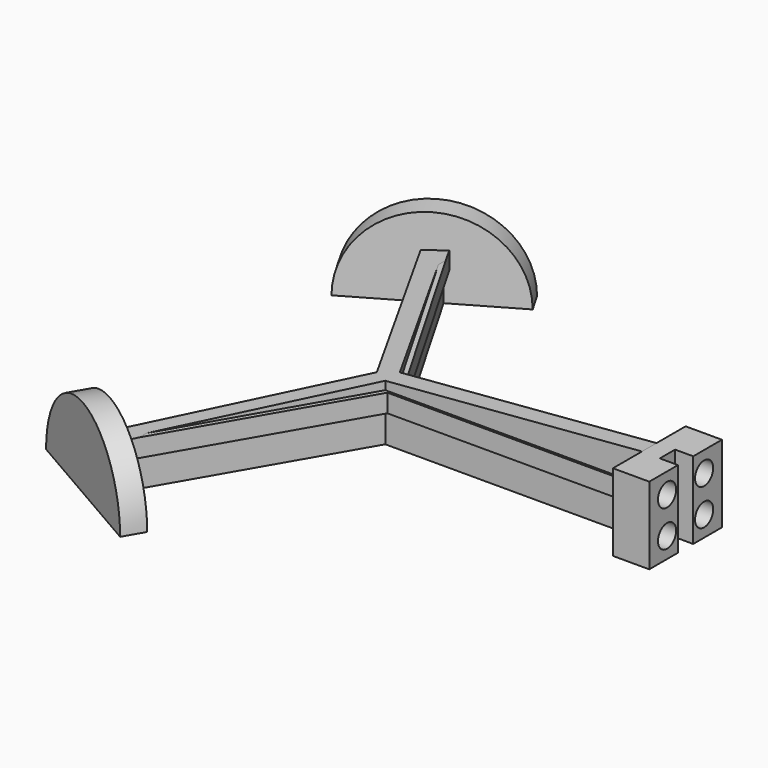
from build123d import *

# Parameters (mm, degrees)
F0_W      = 20
F0_H      = 17
F1_DEPTH  = 8
F2_W      = 4
F2_H      = 4.2
F3_DEPTH  = 17.001
F4_R      = 2.5
F5_DEPTH  = 8.001
F6_W      = 4
F6_H      = 6.5
F6_W_2    = 0.5
F6_H_2    = 4
F7_DEPTH  = 60
F9_DEPTH  = 17.001
F10_DEPTH = 50
F11_DEPTH = 50
F13_DEPTH = 47.8022701892
F14_DEPTH = 43.8022701892
F15_R     = 17.5
F16_DEPTH = 5
F17_R     = 17.5
F18_DEPTH = 5
F20_DEPTH = 108.9243937587


# Not quite as in the source:
# - a feature names something its author has since deleted; it is built from what else it names


with BuildPart() as f1:
    # F0 (on Right) → F1 (new body)
    with BuildSketch(Plane.YZ):
        Rectangle(F0_W, F0_H)
    extrude(amount=F1_DEPTH)

    # F2 (on face) → F3 (cut, through all)
    with BuildSketch(Plane.XY.offset(8.5)):
        with Locations((6, 0)):
            Rectangle(F2_W, F2_H)
    extrude(amount=-F3_DEPTH, mode=Mode.SUBTRACT)

    # F4 (on face) → F5 (cut, through all)
    with BuildSketch(Plane.YZ.offset(8)):
        with Locations((-5.1, 4)):
            Circle(F4_R)
        with Locations((5.1, 4)):
            Circle(F4_R)
        with Locations((-5.1, -4)):
            Circle(F4_R)
        with Locations((5.1, -4)):
            Circle(F4_R)
    extrude(amount=-F5_DEPTH, mode=Mode.SUBTRACT)

    # F6 (on Right) → F7 (join)
    with BuildSketch(Plane.YZ):
        with Locations((0, 5.25)):
            Rectangle(F6_W, F6_H)
        with Locations((2.25, 0)):
            Rectangle(F6_W_2, F6_H_2)
        Rectangle(F6_W, F6_H_2)
        with Locations((-2.25, 0)):
            Rectangle(F6_W_2, F6_H_2)
        with Locations((0, -5.25)):
            Rectangle(F6_W, F6_H)
    extrude(amount=-F7_DEPTH)

    # F8 (on face) → F9 (cut, through all)
    with BuildSketch(Plane.XY.offset(8.5)):
        Polygon((-60, -2.5), (-55.6698729811, -2.5), (-60, 0), align=None)
        Polygon((-60, 2.5), (-60, 0), (-55.6698729811, 2.5), align=None)
    extrude(amount=-F9_DEPTH, mode=Mode.SUBTRACT)

    # F10 (add): a face of the model
    f10_faces = [f1.faces().sort_by_distance(p)[0] for p in [
        (-58.1476678863, -1.0694444444, 0),
    ]]
    extrude(f10_faces, amount=F10_DEPTH)

    # F11 (add): a face of the model
    f11_faces = [f1.faces().sort_by_distance(p)[0] for p in [
        (-58.1476678863, 1.0694444444, 0),
    ]]
    extrude(f11_faces, amount=F11_DEPTH)

    # F12 (on face) → F13 (cut, through all)
    with BuildSketch(Plane.XZ.offset(2)):
        Polygon((0, 8.5), (-90.0749489665, 12.646025978), (-90.0749489665, 1.0502453661), align=None)
    extrude(amount=-F13_DEPTH, mode=Mode.SUBTRACT)

    # F12 (on face) → F14 (cut, through all)
    with BuildSketch(Plane.XZ.offset(2)):
        Polygon((0, 8.5), (-90.0749489665, 12.646025978), (-90.0749489665, 1.0502453661), align=None)
    extrude(amount=F14_DEPTH, mode=Mode.SUBTRACT)

    # F15 (on face) → F16 (join)
    with BuildSketch(Plane(origin=(-40, -69.2820323028, 0), x_dir=(0.8660254038, -0.5, 0), z_dir=(-0.5, -0.8660254038, 0))):
        with Locations((-49.9615242271, -8.5)):
            Circle(F15_R)
    extrude(amount=F16_DEPTH)

    # F17 (on face) → F18 (join)
    with BuildSketch(Plane(origin=(-40, 69.2820323028, 0), x_dir=(-0.8660254038, -0.5, 0), z_dir=(-0.5, 0.8660254038, 0))):
        with Locations((49.9615242271, -8.5)):
            Circle(F17_R)
    extrude(amount=F18_DEPTH)

    # F19 (on face) → F20 (cut, through all)
    with BuildSketch(Plane.YZ.offset(8)):
        Polygon((63.882611692, -8.5), (0, -8.5), (-60.1151846349, -8.5), (-60.0160695612, -29.4797774404), (63.882611692, -28.5877082497), align=None)
    extrude(amount=-F20_DEPTH, mode=Mode.SUBTRACT)


solid = f1.part
